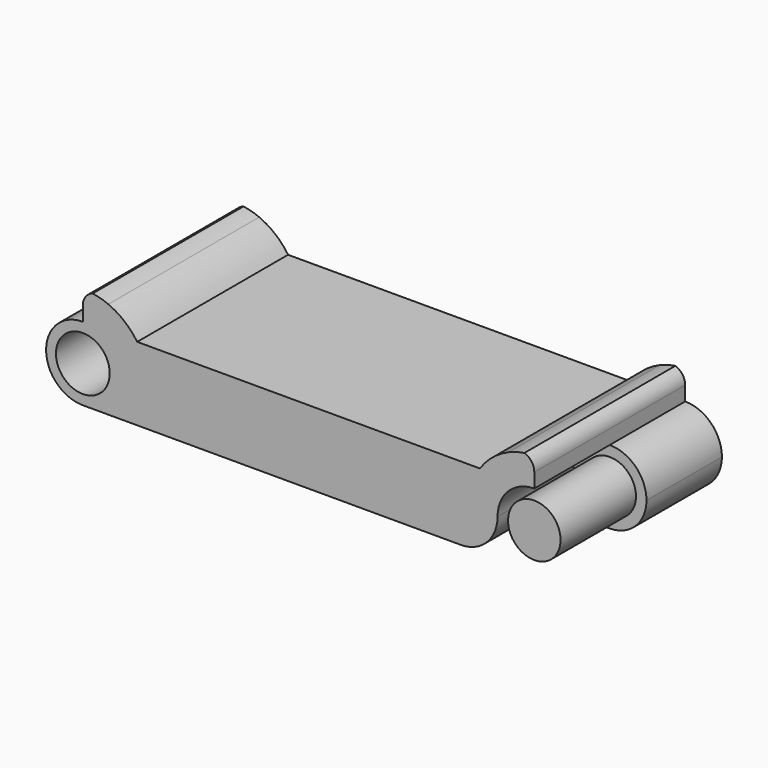
from build123d import *

# Parameters (mm, degrees)
F0_R     = 2
F1_DEPTH = 14.37
F2_DEPTH = 14.37
F3_DEPTH = 7.185
F0_R_2   = 2.05
F4_DEPTH = 14.37


# Not quite as in the source:
# - a feature names something its author has since deleted; it is built from what else it names


with BuildPart() as f1:
    # F0 (on Front) → F1 (new body)
    with BuildSketch(Plane.XZ):
        with Locations((37.2, 2.8)):
            Circle(F0_R)
    extrude(amount=F1_DEPTH)



with BuildPart() as f2:
    # F0 (on Front) → F2 (new body)
    with BuildSketch(Plane.XZ):
        with BuildLine():
            ThreePointArc((5.6, 2.8), (6.4201010127, 0.8201010127), (8.4, 0))
            Line((8.4, 0), (31.6, 0))
            ThreePointArc((31.6, 0), (33.5798989873, 0.8201010127), (34.4, 2.8))
            ThreePointArc((34.4, 2.8), (35.2201010127, 4.7798989873), (37.2, 5.6))
            Line((37.2, 5.6), (37.2, 6.7))
            ThreePointArc((37.2, 6.7), (36.9926506427, 7.3427867688), (36.4487730361, 7.7432436768))
            ThreePointArc((36.4487730361, 7.7432436768), (35.8426991749, 7.6122483799), (35.2574998019, 7.4072435339))
            ThreePointArc((35.2574998019, 7.4072435339), (35.103012566, 6.2352247249), (36.1, 5.6))
            Line((36.1, 5.6), (33.0575369646, 5.6))
            Line((33.0575369646, 5.6), (6.9424630354, 5.6))
            Line((6.9424630354, 5.6), (3.9, 5.6))
            ThreePointArc((3.9, 5.6), (4.896987434, 6.2352247249), (4.7425001981, 7.4072435339))
            ThreePointArc((4.7425001981, 7.4072435339), (4.1573008251, 7.6122483799), (3.5512269639, 7.7432436768))
            ThreePointArc((3.5512269639, 7.7432436768), (3.0073493573, 7.3427867688), (2.8, 6.7))
            Line((2.8, 6.7), (2.8, 5.6))
            ThreePointArc((2.8, 5.6), (4.7798989873, 4.7798989873), (5.6, 2.8))
        make_face()
        with BuildLine():
            ThreePointArc((35.2574998019, 7.4072435339), (34.0261653027, 6.6635182559), (33.0575369646, 5.6))
            Line((33.0575369646, 5.6), (36.1, 5.6))
            ThreePointArc((36.1, 5.6), (35.103012566, 6.2352247249), (35.2574998019, 7.4072435339))
        make_face()
        with BuildLine():
            ThreePointArc((6.9424630354, 5.6), (5.9738346973, 6.6635182559), (4.7425001981, 7.4072435339))
            ThreePointArc((4.7425001981, 7.4072435339), (4.896987434, 6.2352247249), (3.9, 5.6))
            Line((3.9, 5.6), (6.9424630354, 5.6))
        make_face()
    extrude(amount=F2_DEPTH)


with BuildPart() as f1_1:
    add(f1.part)

    add(f2.part)  # F3 merges F2
    # F0 (on Front) → F3 (join)
    with BuildSketch(Plane.XZ):
        with BuildLine():
            ThreePointArc((34.4, 2.8), (35.2201010127, 0.8201010127), (37.2, 0))
            ThreePointArc((37.2, 0), (39.1798989873, 0.8201010127), (40, 2.8))
            ThreePointArc((40, 2.8), (39.1798989873, 4.7798989873), (37.2, 5.6))
            ThreePointArc((37.2, 5.6), (35.2201010127, 4.7798989873), (34.4, 2.8))
        make_face()
        with Locations((37.2, 2.8)):
            Circle(F0_R, mode=Mode.SUBTRACT)
        with BuildLine():
            ThreePointArc((34.4, 2.8), (33.5798989873, 0.8201010127), (31.6, 0))
            Line((31.6, 0), (37.2, 0))
            ThreePointArc((37.2, 0), (35.2201010127, 0.8201010127), (34.4, 2.8))
        make_face()
    extrude(amount=F3_DEPTH)

    # F0 (on Front) → F4 (join)
    with BuildSketch(Plane.XZ):
        with BuildLine():
            ThreePointArc((5.6, 2.8), (4.7798989873, 0.8201010127), (2.8, 0))
            Line((2.8, 0), (8.4, 0))
            ThreePointArc((8.4, 0), (6.4201010127, 0.8201010127), (5.6, 2.8))
        make_face()
        with BuildLine():
            ThreePointArc((2.8, 5.6), (0, 2.8), (2.8, 0))
            ThreePointArc((2.8, 0), (4.7798989873, 0.8201010127), (5.6, 2.8))
            ThreePointArc((5.6, 2.8), (4.7798989873, 4.7798989873), (2.8, 5.6))
        make_face()
        with Locations((2.8, 2.8)):
            Circle(F0_R_2, mode=Mode.SUBTRACT)
    extrude(amount=F4_DEPTH)


solid = f1_1.part
